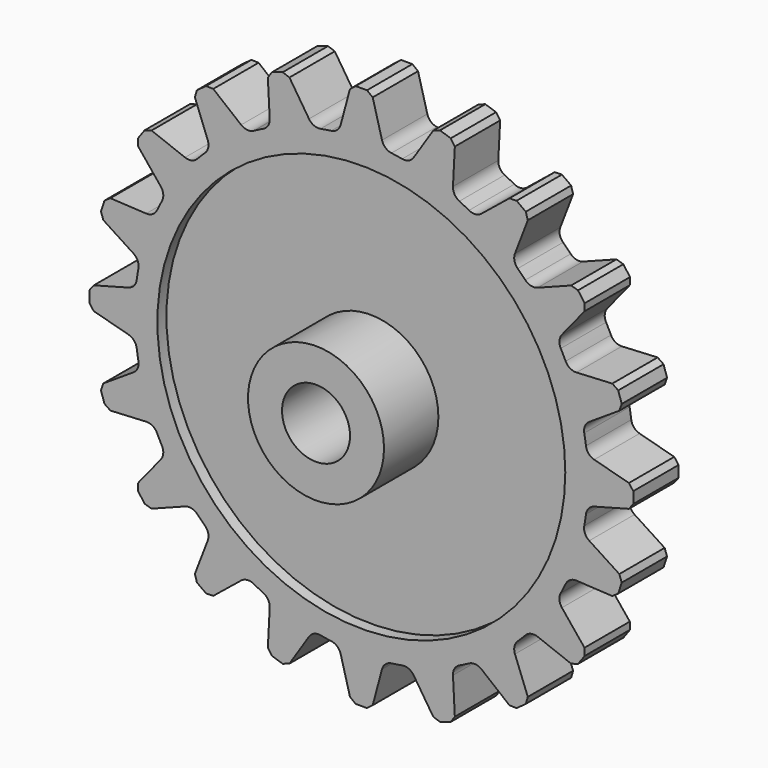
from build123d import *

# Parameters (mm, degrees)
F0_R            = 100
F1_DEPTH        = 25
F3_DEPTH        = 25
F3_COPIES_COUNT = 20
F4_SIZE         = 2
F5_R            = 5
F6_R            = 90
F7_DEPTH        = 5
F8_R            = 30
F8_R_2          = 15
F9_DEPTH        = 30


# Not quite as in the source:
# - a pattern or mirror of a feature is missing from the dataset's text; its kind, count and spacing are read off the source's solid


with BuildPart() as f1:
    # F0 (on Front) → F1 (new body)
    with BuildSketch(Plane.XZ):
        Circle(F0_R)
    extrude(amount=F1_DEPTH)

    # F2 (on face) → F3 (join)
    with BuildSketch(Plane.XZ.offset(25)):
        Polygon((-4.5, 120), (-9.9931095726, 99.4994359837), (9.9931095726, 99.4994359837), (4.5, 120), align=None)
    f3 = extrude(amount=-F3_DEPTH)

    # F3_copies: F3 ×20 about axis
    f3_copies_axis = Axis((0, 0, 0), (0, 1, 0))
    for i in range(1, F3_COPIES_COUNT):
        add(f3.rotate(f3_copies_axis, i * 360 / F3_COPIES_COUNT))

    # F4
    f4_edges = [f1.edges().sort_by_distance(p)[0] for p in [
        (4.5, -12.5, 120),
        (-4.5, -12.5, 120),
        (-32.802285, -12.5, 115.517358),
        (115.517358, -12.5, 32.802285),
        (120, -12.5, 4.5),
        (120, -12.5, -4.5),
        (115.517358, -12.5, -32.802285),
        (112.736205, -12.5, -41.361794),
        (99.727073, -12.5, -66.893654),
        (94.437006, -12.5, -74.174807),
        (74.174807, -12.5, -94.437006),
        (66.893654, -12.5, -99.727073),
        (41.361794, -12.5, -112.736205),
        (32.802285, -12.5, -115.517358),
        (4.5, -12.5, -120),
        (-4.5, -12.5, -120),
        (-32.802285, -12.5, -115.517358),
        (-41.361794, -12.5, -112.736205),
        (-66.893654, -12.5, -99.727073),
        (-74.174807, -12.5, -94.437006),
        (-94.437006, -12.5, -74.174807),
        (-99.727073, -12.5, -66.893654),
        (-112.736205, -12.5, -41.361794),
        (-115.517358, -12.5, -32.802285),
        (-120, -12.5, -4.5),
        (-120, -12.5, 4.5),
        (-115.517358, -12.5, 32.802285),
        (-112.736205, -12.5, 41.361794),
        (-99.727073, -12.5, 66.893654),
        (-94.437006, -12.5, 74.174807),
        (-74.174807, -12.5, 94.437006),
        (-66.893654, -12.5, 99.727073),
        (32.802285, -12.5, 115.517358),
        (41.361794, -12.5, 112.736205),
        (66.893654, -12.5, 99.727073),
        (74.174807, -12.5, 94.437006),
        (94.437006, -12.5, 74.174807),
        (99.727073, -12.5, 66.893654),
        (112.736205, -12.5, 41.361794),
        (-41.361794, -12.5, 112.736205),
    ]]
    chamfer(f4_edges, length=F4_SIZE)

    # F5
    f5_edges = [f1.edges().sort_by_distance(p)[0] for p in [
        (9.99311, -12.5, 99.499436),
        (-9.99311, -12.5, 99.499436),
        (97.717628, -12.5, 21.243005),
        (99.499436, -12.5, 9.99311),
        (91.541546, -12.5, 40.251029),
        (86.370537, -12.5, 50.399706),
        (99.499436, -12.5, -9.99311),
        (97.717628, -12.5, -21.243005),
        (74.622932, -12.5, 66.568897),
        (66.568897, -12.5, 74.622932),
        (91.541546, -12.5, -40.251029),
        (86.370537, -12.5, -50.399706),
        (50.399706, -12.5, 86.370537),
        (40.251029, -12.5, 91.541546),
        (74.622932, -12.5, -66.568897),
        (66.568897, -12.5, -74.622932),
        (21.243005, -12.5, 97.717628),
        (50.399706, -12.5, -86.370537),
        (40.251029, -12.5, -91.541546),
        (-21.243005, -12.5, 97.717628),
        (21.243005, -12.5, -97.717628),
        (9.99311, -12.5, -99.499436),
        (-40.251029, -12.5, 91.541546),
        (-50.399706, -12.5, 86.370537),
        (-9.99311, -12.5, -99.499436),
        (-21.243005, -12.5, -97.717628),
        (-66.568897, -12.5, 74.622932),
        (-74.622932, -12.5, 66.568897),
        (-40.251029, -12.5, -91.541546),
        (-50.399706, -12.5, -86.370537),
        (-86.370537, -12.5, 50.399706),
        (-91.541546, -12.5, 40.251029),
        (-66.568897, -12.5, -74.622932),
        (-74.622932, -12.5, -66.568897),
        (-97.717628, -12.5, 21.243005),
        (-99.499436, -12.5, 9.99311),
        (-86.370537, -12.5, -50.399706),
        (-91.541546, -12.5, -40.251029),
        (-99.499436, -12.5, -9.99311),
        (-97.717628, -12.5, -21.243005),
    ]]
    fillet(f5_edges, radius=F5_R)

    # F6 (on face) → F7 (cut)
    with BuildSketch(Plane.XZ.offset(25)):
        Circle(F6_R)
    extrude(amount=-F7_DEPTH, mode=Mode.SUBTRACT)

    # F8 (on face) → F9 (join)
    with BuildSketch(Plane.XZ.offset(20)):
        Circle(F8_R)
        Circle(F8_R_2, mode=Mode.SUBTRACT)
    extrude(amount=F9_DEPTH)


solid = f1.part
